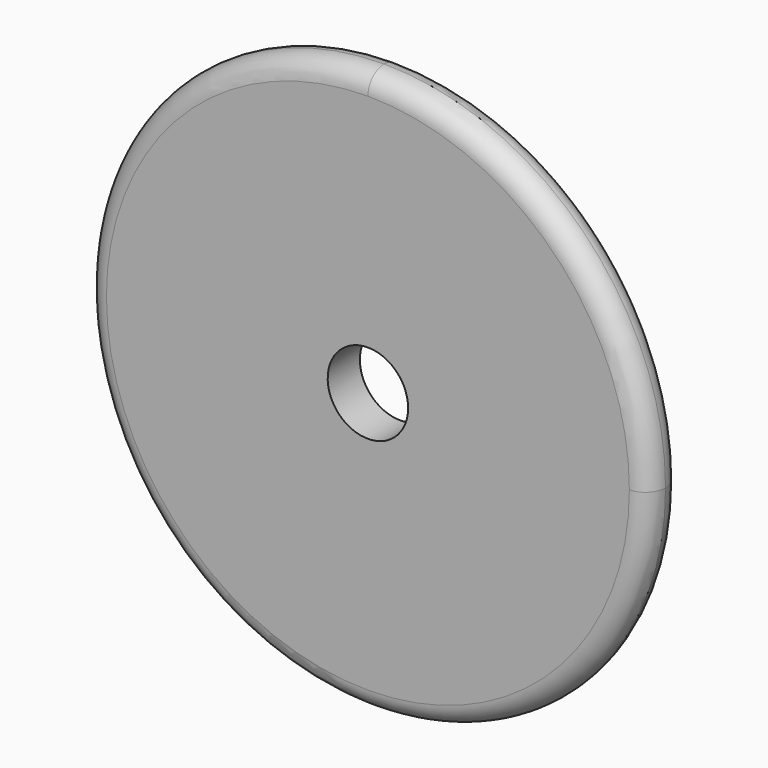
from build123d import *

# Parameters (mm, degrees)
F1_DEPTH = 10
F2_R     = 4.99999


# Not quite as in the source:
# - a fillet or chamfer is up to 0.001 mm smaller than in the source, because OpenCascade refuses the exact size


with BuildPart() as f1:
    # F0 (on Front) → F1 (new body)
    with BuildSketch(Plane.XZ):
        with BuildLine():
            ThreePointArc((0, 70), (-49.4974746831, -49.4974746831), (70, 0))
            ThreePointArc((70, 0), (49.4974746831, 49.4974746831), (0, 70))
        make_face()
        with BuildLine():
            ThreePointArc((10, 0), (-7.0710678119, -7.0710678119), (0, 10))
            ThreePointArc((0, 10), (7.0710678119, 7.0710678119), (10, 0))
        make_face(mode=Mode.SUBTRACT)
    extrude(amount=F1_DEPTH)

    # F2 (radius 5 in the source; OpenCascade refuses exactly that, so slightly less here)
    f2_edges = [f1.edges().sort_by_distance(p)[0] for p in [
        (-70, -10, 0),
        (-70, 0, 0),
    ]]
    fillet(f2_edges, radius=F2_R)


solid = f1.part
